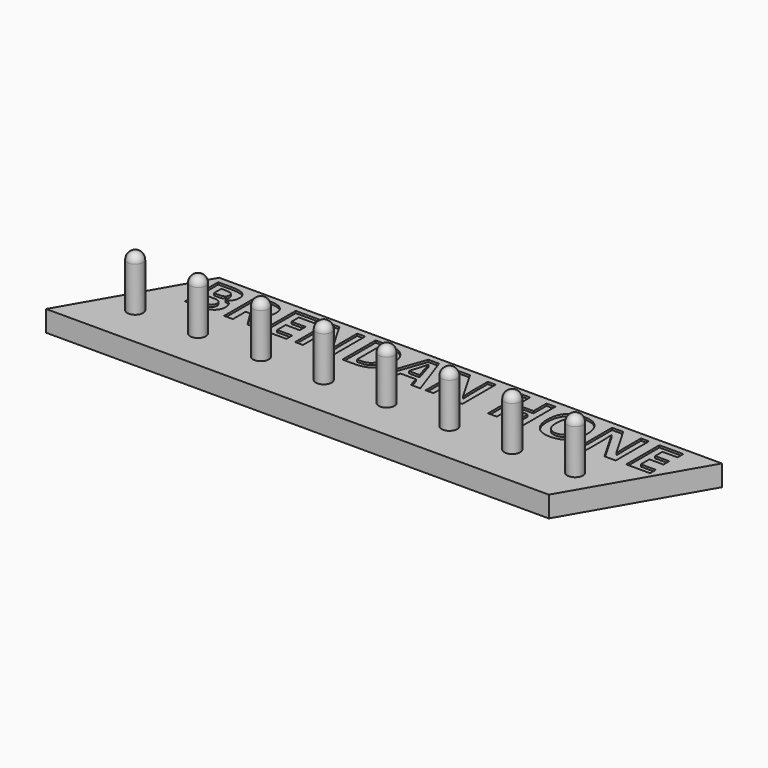
from build123d import *

# Parameters (mm, degrees)
F1_DEPTH     = 25.4
F2_R         = 9.525
F3_DEPTH     = 63.5
F4_R         = 9.525
F5_TEXT_SIZE = 70.5555555556
F6_DEPTH     = 2.54


# Not quite as in the source:
# - Text() gives the source's letters only with a copy of the font that has no kerning and outlines rounded to 1/6400 em; it was checked with that copy


with BuildPart() as f1:
    # F0 (on Top) → F1 (new body)
    with BuildSketch(Plane.XY):
        Polygon((87.98814, 152.3999289435), (0, 0), (609.6, 0), (697.58814, 152.3999289435), align=None)
    extrude(amount=F1_DEPTH)

    # F2 (on face) → F3 (join)
    with BuildSketch(Plane.XY.offset(25.4)):
        with Locations((67.43446, 50.8)):
            Circle(F2_R)
        with Locations((143.63446, 50.8)):
            Circle(F2_R)
        with Locations((219.83446, 50.8)):
            Circle(F2_R)
        with Locations((296.03446, 50.8)):
            Circle(F2_R)
        with Locations((372.23446, 50.8)):
            Circle(F2_R)
        with Locations((448.43446, 50.8)):
            Circle(F2_R)
        with Locations((524.63446, 50.8)):
            Circle(F2_R)
        with Locations((600.83446, 50.8)):
            Circle(F2_R)
    extrude(amount=F3_DEPTH)

    # F4
    f4_edges = [f1.edges().sort_by_distance(p)[0] for p in [
        (57.90946, 50.8, 88.9),
        (134.10946, 50.8, 88.9),
        (210.30946, 50.8, 88.9),
        (286.50946, 50.8, 88.9),
        (362.70946, 50.8, 88.9),
        (438.90946, 50.8, 88.9),
        (515.10946, 50.8, 88.9),
        (591.30946, 50.8, 88.9),
    ]]
    fillet(f4_edges, radius=F4_R)

    # F5 (on face) → F6 (cut)
    with BuildSketch(Plane.XY.offset(25.4)):
        with Locations((86.6877250373, 94.2477391481)):
            Text('BRENDAN HONE', F5_TEXT_SIZE, font='Open Sans', font_style=FontStyle.BOLD, text_align=(TextAlign.LEFT, TextAlign.BOTTOM))
    extrude(amount=-F6_DEPTH, mode=Mode.SUBTRACT)


solid = f1.part
